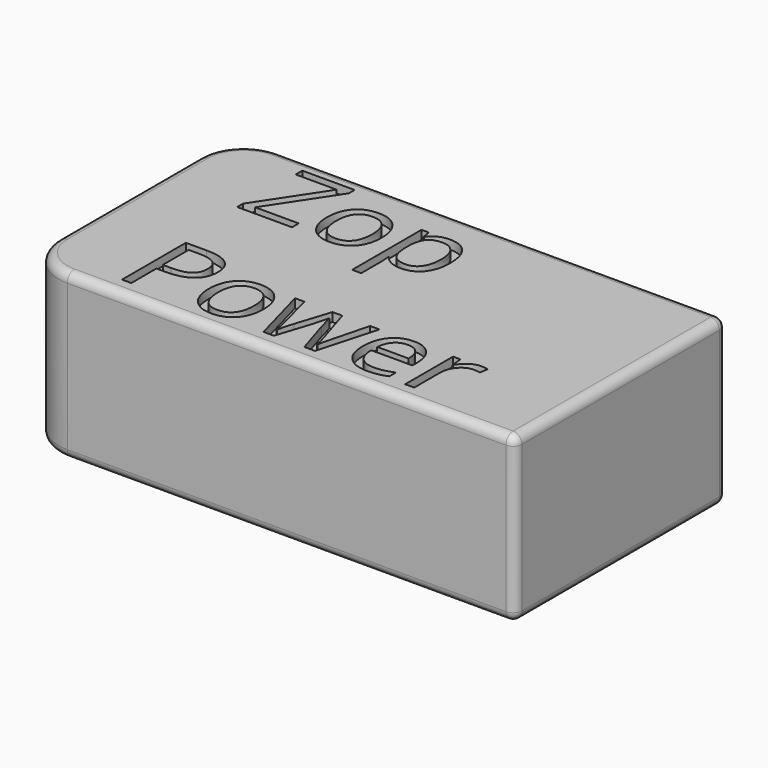
from build123d import *

# Parameters (mm, degrees)
F0_W         = 55.4
F0_H         = 29.8
F1_DEPTH     = 9.25
F2_R         = 5
F3_R         = 1
F4_TEXT_SIZE = 12.5915672268
F5_DEPTH     = 1


# Not quite as in the source:
# - Text() gives the source's letters only with a copy of the font that has no kerning and outlines rounded to 1/6400 em; it was checked with that copy


with BuildPart() as f1:
    # F0 (on Top) → F1 (new body, symmetric)
    with BuildSketch(Plane.XY):
        Rectangle(F0_W, F0_H)
    extrude(amount=F1_DEPTH, both=True)

    # F2
    f2_edges = [f1.edges().sort_by_distance(p)[0] for p in [
        (-27.7, 14.9, 0),
        (-27.7, -14.9, 0),
    ]]
    fillet(f2_edges, radius=F2_R)

    # F3
    f3_edges = [f1.edges().sort_by_distance(p)[0] for p in [
        (2.5, 14.9, 9.25),
        (-26.235534, 13.435534, 9.25),
        (27.7, 0, 9.25),
        (-27.7, 0, 9.25),
        (2.5, -14.9, 9.25),
        (-26.235534, -13.435534, 9.25),
        (2.5, 14.9, -9.25),
        (-26.235534, 13.435534, -9.25),
        (27.7, 0, -9.25),
        (-27.7, 0, -9.25),
        (2.5, -14.9, -9.25),
        (-26.235534, -13.435534, -9.25),
        (27.7, 14.9, 0),
        (27.7, -14.9, 0),
    ]]
    fillet(f3_edges, radius=F3_R)

    # F4 (on face) → F5 (cut)
    with BuildSketch(Plane.XY.offset(9.25)):
        with Locations((-19.4042660296, 4.2546256445)):
            Text('Zop', F4_TEXT_SIZE, font='Open Sans', text_align=(TextAlign.LEFT, TextAlign.BOTTOM))
        with Locations((-19.4042660296, -12.8699057839)):
            Text('Power', F4_TEXT_SIZE, font='Open Sans', text_align=(TextAlign.LEFT, TextAlign.BOTTOM))
    extrude(amount=-F5_DEPTH, mode=Mode.SUBTRACT)


solid = f1.part
